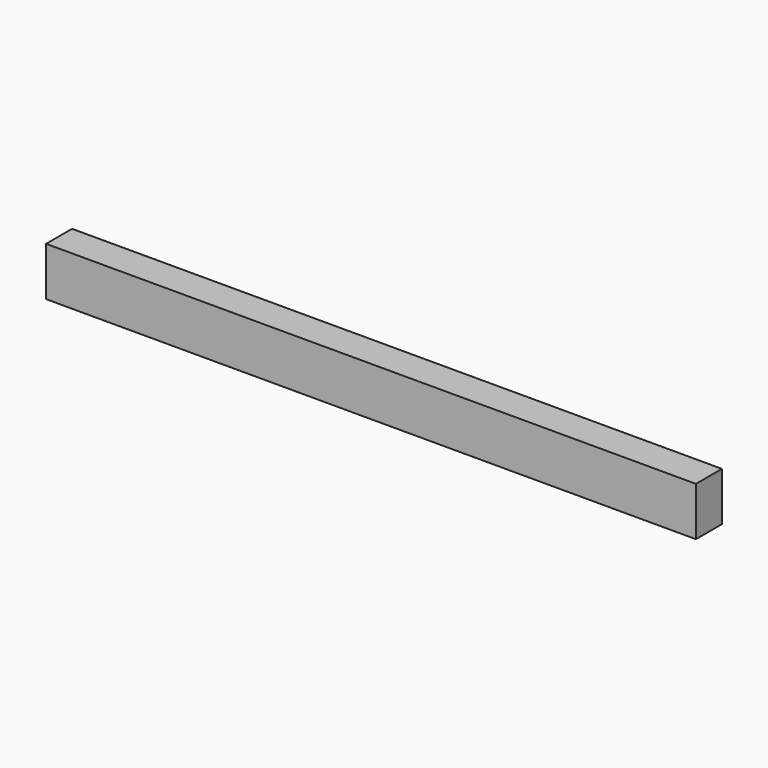
from build123d import *

# Parameters (mm, degrees)
F0_W     = 254
F0_H     = 19.05
F1_DEPTH = 12.7


# Not quite as in the source:
# - a feature names something its author has since deleted; it is built from what else it names


with BuildPart() as f1:
    # F0 (on Front) → F1 (new body)
    with BuildSketch(Plane.XZ):
        with Locations((66.0400510788, 144.9867119074)):
            Rectangle(F0_W, F0_H)
    extrude(amount=F1_DEPTH)


solid = f1.part
